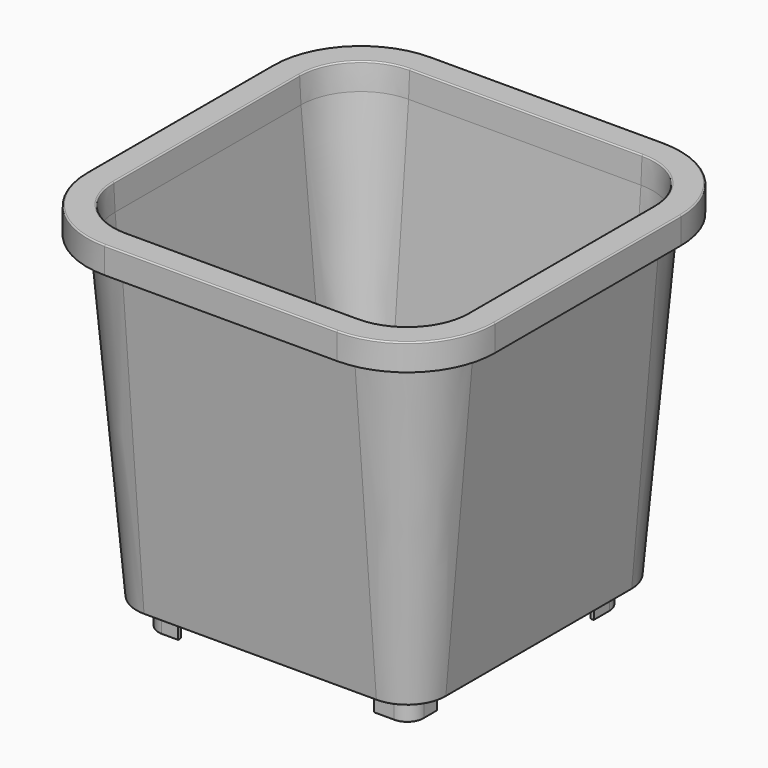
from build123d import *

# Parameters (mm, degrees)
F1_DEPTH = 4
F1_TAPER = -3
F2_DEPTH = 48
F2_TAPER = 5
F3_T     = 1
F5_DEPTH = 4
F7_DEPTH = 3
F9_DEPTH = 4
F10_R    = 0.2


# Not quite as in the source:
# - a shell that OpenCascade refuses in one call is made with other operations: the cavity is built on its own and cut out


with BuildPart() as f1:
    # F0 (on Top) → F1 (new body)
    with BuildSketch(Plane.XY):
        with BuildLine():
            Line((-17.5, -27.5), (17.5, -27.5))
            ThreePointArc((17.5, -27.5), (24.5710678119, -24.5710678119), (27.5, -17.5))
            Line((27.5, -17.5), (27.5, 17.5))
            ThreePointArc((27.5, 17.5), (24.5710678119, 24.5710678119), (17.5, 27.5))
            Line((17.5, 27.5), (-17.5, 27.5))
            ThreePointArc((-17.5, 27.5), (-24.5710678119, 24.5710678119), (-27.5, 17.5))
            Line((-27.5, 17.5), (-27.5, -17.5))
            ThreePointArc((-27.5, -17.5), (-24.5710678119, -24.5710678119), (-17.5, -27.5))
        make_face()
    extrude(amount=F1_DEPTH, taper=F1_TAPER)

    # F1_face (on face) → F2 (join)
    with BuildSketch(Plane(origin=(0, 0, 0), x_dir=(1, 0, 0), z_dir=(0, 0, -1))):
        with BuildLine():
            ThreePointArc((-17.5, 27.5), (-24.5710678119, 24.5710678119), (-27.5, 17.5))
            Line((-27.5, 17.5), (-27.5, -17.5))
            ThreePointArc((-27.5, -17.5), (-24.5710678119, -24.5710678119), (-17.5, -27.5))
            Line((-17.5, -27.5), (17.5, -27.5))
            ThreePointArc((17.5, -27.5), (24.5710678119, -24.5710678119), (27.5, -17.5))
            Line((27.5, -17.5), (27.5, 17.5))
            ThreePointArc((27.5, 17.5), (24.5710678119, 24.5710678119), (17.5, 27.5))
            Line((17.5, 27.5), (-17.5, 27.5))
        make_face()
    extrude(amount=F2_DEPTH, taper=F2_TAPER)

    # F3: shell of thickness 1, made by hand


with BuildPart() as f3_core1:
    # F3_t2: copy of F1
    add(f1.part)

    # the walls: a layer under each face that stays
    f3_faces = [f3_core1.faces().sort_by_distance(p)[0] for p in [
        (-24.6451836041, -24.6451836041, 2),
        (-23.0863359577, -23.0863359577, -24),
        (0, -27.6048155586, 2),
        (-27.6048155586, 0, 2),
        (-25.4002720754, 0, -24),
        (0, 0, -48),
        (0, -25.4002720754, -24),
        (24.6451836041, -24.6451836041, 2),
        (27.6048155586, 0, 2),
        (24.6451836041, 24.6451836041, 2),
        (0, 27.6048155586, 2),
        (-24.6451836041, 24.6451836041, 2),
        (-23.0863359577, 23.0863359577, -24),
        (0, 25.4002720754, -24),
        (23.0863359577, 23.0863359577, -24),
        (25.4002720754, 0, -24),
        (23.0863359577, -23.0863359577, -24),
    ]]
    thicken(f3_faces, amount=-F3_T, mode=Mode.SUBTRACT)


with BuildPart() as f1_1:
    add(f1.part)

    # what is left inside the walls is the cavity
    f3_cavity = [f3_core1.part.solids().sort_by_distance(p)[0] for p in [
        (0, 8.902753, 3.99),
    ]]
    add(f3_cavity, mode=Mode.SUBTRACT)

    # F4 (on face) → F5 (join)
    with BuildSketch(Plane.XY.offset(4)):
        with BuildLine():
            ThreePointArc((30.7096311171, 17.5), (26.8406197399, 26.8406197399), (17.5, 30.7096311171))
            Line((17.5, 30.7096311171), (-17.5, 30.7096311171))
            ThreePointArc((-17.5, 30.7096311171), (-26.8406197399, 26.8406197399), (-30.7096311171, 17.5))
            Line((-30.7096311171, 17.5), (-30.7096311171, -17.5))
            ThreePointArc((-30.7096311171, -17.5), (-26.8406197399, -26.8406197399), (-17.5, -30.7096311171))
            Line((-17.5, -30.7096311171), (17.5, -30.7096311171))
            ThreePointArc((17.5, -30.7096311171), (26.8406197399, -26.8406197399), (30.7096311171, -17.5))
            Line((30.7096311171, -17.5), (30.7096311171, 17.5))
        make_face()
        with BuildLine():
            ThreePointArc((-26.7082587711, 17.5), (-24.01122222, 24.01122222), (-17.5, 26.7082587711))
            Line((-17.5, 26.7082587711), (17.5, 26.7082587711))
            ThreePointArc((17.5, 26.7082587711), (24.01122222, 24.01122222), (26.7082587711, 17.5))
            Line((26.7082587711, 17.5), (26.7082587711, -17.5))
            ThreePointArc((26.7082587711, -17.5), (24.01122222, -24.01122222), (17.5, -26.7082587711))
            Line((17.5, -26.7082587711), (-17.5, -26.7082587711))
            ThreePointArc((-17.5, -26.7082587711), (-24.01122222, -24.01122222), (-26.7082587711, -17.5))
            Line((-26.7082587711, -17.5), (-26.7082587711, 17.5))
        make_face(mode=Mode.SUBTRACT)
    extrude(amount=-F5_DEPTH)

    # F6 (on face) → F7 (cut)
    with BuildSketch(Plane(origin=(0, 0, 0), x_dir=(1, 0, 0), z_dir=(0, 0, -1))):
        with BuildLine():
            ThreePointArc((-17.5, 29.7096311171), (-26.1335129587, 26.1335129587), (-29.7096311171, 17.5))
            Line((-29.7096311171, 17.5), (-29.7096311171, -17.5))
            ThreePointArc((-29.7096311171, -17.5), (-26.1335129587, -26.1335129587), (-17.5, -29.7096311171))
            Line((-17.5, -29.7096311171), (17.5, -29.7096311171))
            ThreePointArc((17.5, -29.7096311171), (26.1335129587, -26.1335129587), (29.7096311171, -17.5))
            Line((29.7096311171, -17.5), (29.7096311171, 17.5))
            ThreePointArc((29.7096311171, 17.5), (26.1335129587, 26.1335129587), (17.5, 29.7096311171))
            Line((17.5, 29.7096311171), (-17.5, 29.7096311171))
        make_face()
        with BuildLine():
            Line((-27.5, -17.5), (-27.5, 17.5))
            ThreePointArc((-27.5, 17.5), (-24.5710678119, 24.5710678119), (-17.5, 27.5))
            Line((-17.5, 27.5), (17.5, 27.5))
            ThreePointArc((17.5, 27.5), (24.5710678119, 24.5710678119), (27.5, 17.5))
            Line((27.5, 17.5), (27.5, -17.5))
            ThreePointArc((27.5, -17.5), (24.5710678119, -24.5710678119), (17.5, -27.5))
            Line((17.5, -27.5), (-17.5, -27.5))
            ThreePointArc((-17.5, -27.5), (-24.5710678119, -24.5710678119), (-27.5, -17.5))
        make_face(mode=Mode.SUBTRACT)
    extrude(amount=-F7_DEPTH, mode=Mode.SUBTRACT)

    # F8 (on face) → F9 (join)
    with BuildSketch(Plane(origin=(0, 0, -48), x_dir=(1, 0, 0), z_dir=(0, 0, -1))):
        with BuildLine():
            Line((-15, 19.5), (-15, 20))
            Line((-15, 20), (-17.5, 20))
            ThreePointArc((-17.5, 20), (-19.267766953, 19.267766953), (-20, 17.5))
            Line((-20, 17.5), (-20, 14.5))
            Line((-20, 14.5), (-19.5, 14.5))
            Line((-19.5, 14.5), (-19.5, 17.5))
            ThreePointArc((-19.5, 17.5), (-18.9142135624, 18.9142135624), (-17.5, 19.5))
            Line((-17.5, 19.5), (-15, 19.5))
        make_face()
        with BuildLine():
            Line((19.5000000696, 17.4999999225), (19.5000000596, 14.9999999225))
            Line((19.5000000596, 14.9999999225), (20.0000000596, 14.9999999205))
            Line((20.0000000596, 14.9999999205), (20.0000000696, 17.4999999205))
            ThreePointArc((20.0000000696, 17.4999999205), (19.2677670296, 19.2677668764), (17.5000000795, 19.9999999304))
            Line((17.5000000795, 19.9999999304), (14.5000000795, 19.9999999424))
            Line((14.5000000795, 19.9999999424), (14.5000000775, 19.4999999424))
            Line((14.5000000775, 19.4999999424), (17.5000000775, 19.4999999304))
            ThreePointArc((17.5000000775, 19.4999999304), (18.9142136376, 18.9142134872), (19.5000000696, 17.4999999225))
        make_face()
        with BuildLine():
            Line((17.499999845, -19.5000001391), (14.999999845, -19.5000001192))
            Line((14.999999845, -19.5000001192), (14.999999841, -20.0000001192))
            Line((14.999999841, -20.0000001192), (17.499999841, -20.0000001391))
            ThreePointArc((17.499999841, -20.0000001391), (19.2677667998, -19.2677671061), (19.9999998609, -17.500000159))
            Line((19.9999998609, -17.500000159), (19.9999998847, -14.500000159))
            Line((19.9999998847, -14.500000159), (19.4999998847, -14.500000155))
            Line((19.4999998847, -14.500000155), (19.4999998609, -17.500000155))
            ThreePointArc((19.4999998609, -17.500000155), (18.914213412, -18.9142137127), (17.499999845, -19.5000001391))
        make_face()
        with BuildLine():
            Line((-19.5000002087, -17.4999997675), (-19.5000001789, -14.9999997675))
            Line((-19.5000001789, -14.9999997675), (-20.0000001789, -14.9999997615))
            Line((-20.0000001789, -14.9999997615), (-20.0000002087, -17.4999997615))
            ThreePointArc((-20.0000002087, -17.4999997615), (-19.2677671827, -19.2677667232), (-17.5000002385, -19.9999997913))
            Line((-17.5000002385, -19.9999997913), (-14.5000002385, -19.9999998271))
            Line((-14.5000002385, -19.9999998271), (-14.5000002325, -19.4999998271))
            Line((-14.5000002325, -19.4999998271), (-17.5000002325, -19.4999997913))
            ThreePointArc((-17.5000002325, -19.4999997913), (-18.9142137879, -18.9142133368), (-19.5000002087, -17.4999997675))
        make_face()
    extrude(amount=F9_DEPTH)

    # F10
    f10_edges = [f1_1.edges().sort_by_distance(p)[0] for p in [
        (0, -22.384213, -47),
        (20.95366, -20.95366, -47),
        (22.384213, 0, -47),
        (20.95366, 20.95366, -47),
        (0, 22.384213, -47),
        (-20.95366, 20.95366, -47),
        (-22.384213, 0, -47),
        (-20.95366, -20.95366, -47),
        (-21.601604, -21.601604, -48),
        (0, -23.300544, -48),
        (-23.300544, 0, -48),
        (21.601604, -21.601604, -48),
        (-21.601604, 21.601604, -48),
        (23.300544, 0, -48),
        (0, 23.300544, -48),
        (21.601604, 21.601604, -48),
        (16.25, 19.5, -48),
        (15, 19.75, -48),
        (16.25, 20, -48),
        (19.267767, 19.267767, -48),
        (20, 16, -48),
        (19.75, 14.5, -48),
        (19.5, 16, -48),
        (18.914213, 18.914214, -48),
        (16, -20, -48),
        (14.5, -19.75, -48),
        (16, -19.5, -48),
        (18.914214, -18.914213, -48),
        (19.5, -16.25, -48),
        (19.75, -15, -48),
        (20, -16.25, -48),
        (19.267767, -19.267767, -48),
        (-16, 20, -48),
        (-14.5, 19.75, -48),
        (-16, 19.5, -48),
        (-18.914214, 18.914213, -48),
        (-19.5, 16.25, -48),
        (-19.75, 15, -48),
        (-20, 16.25, -48),
        (-19.267767, 19.267767, -48),
        (-15, -19.75, -48),
        (-16.25, -20, -48),
        (-19.267767, -19.267767, -48),
        (-20, -16, -48),
        (-19.75, -14.5, -48),
        (-19.5, -16, -48),
        (-18.914214, -18.914214, -48),
        (-16.25, -19.5, -48),
        (0, -29.709631, 3),
        (-26.133513, -26.133513, 3),
        (-29.709631, 0, 3),
        (-26.133513, 26.133513, 3),
        (0, 29.709631, 3),
        (26.133513, 26.133513, 3),
        (29.709631, 0, 3),
        (26.133513, -26.133513, 3),
        (-27.5, 0, 3),
        (-24.571068, -24.571068, 3),
        (0, -27.5, 3),
        (24.571068, -24.571068, 3),
        (27.5, 0, 3),
        (24.571068, 24.571068, 3),
        (0, 27.5, 3),
        (-24.571068, 24.571068, 3),
        (-24.011222, -24.011222, 4),
        (-26.708259, 0, 4),
        (-24.011222, 24.011222, 4),
        (0, 26.708259, 4),
        (24.011222, 24.011222, 4),
        (26.708259, 0, 4),
        (24.011222, -24.011222, 4),
        (0, -26.708259, 4),
        (26.84062, 26.84062, 4),
        (0, 30.709631, 4),
        (-26.84062, 26.84062, 4),
        (-30.709631, 0, 4),
        (-26.84062, -26.84062, 4),
        (0, -30.709631, 4),
        (26.84062, -26.84062, 4),
        (30.709631, 0, 4),
        (-16, 20, -52),
        (-14.5, 19.75, -52),
        (-16, 19.5, -52),
        (-18.914214, 18.914213, -52),
        (-19.5, 16.25, -52),
        (-19.75, 15, -52),
        (-20, 16.25, -52),
        (-19.267767, 19.267767, -52),
        (-15, -19.75, -52),
        (-16.25, -20, -52),
        (-19.267767, -19.267767, -52),
        (-20, -16, -52),
        (-19.75, -14.5, -52),
        (-19.5, -16, -52),
        (-18.914214, -18.914214, -52),
        (-16.25, -19.5, -52),
        (16, -20, -52),
        (14.5, -19.75, -52),
        (16, -19.5, -52),
        (18.914214, -18.914213, -52),
        (19.5, -16.25, -52),
        (19.75, -15, -52),
        (20, -16.25, -52),
        (19.267767, -19.267767, -52),
        (16.25, 19.5, -52),
        (15, 19.75, -52),
        (16.25, 20, -52),
        (19.267767, 19.267767, -52),
        (20, 16, -52),
        (19.75, 14.5, -52),
        (19.5, 16, -52),
        (18.914213, 18.914214, -52),
    ]]
    fillet(f10_edges, radius=F10_R)


solid = f1_1.part
